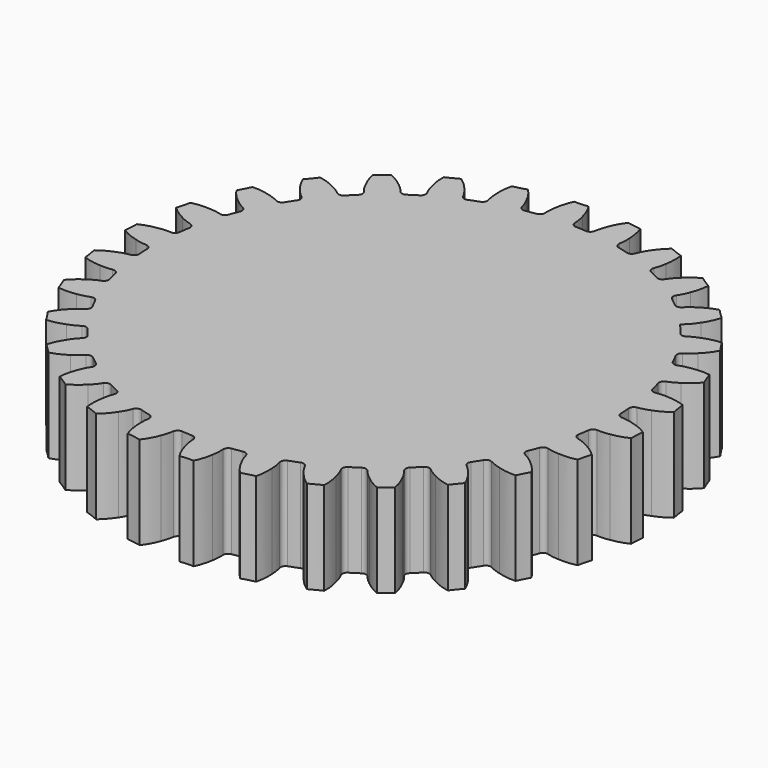
from build123d import *

# Parameters (mm, degrees)
F1_DEPTH = 19.05
F2_COUNT = 30
F4_R     = 1.016


with BuildPart() as f1:
    # F0 (on Top) → F1 (new body)
    with BuildSketch(Plane.XY):
        with BuildLine():
            ThreePointArc((-5.3628156149, 47.1048083691), (-31.5703698192, -35.3685525897), (47.4091, 0))
            ThreePointArc((47.4091, 0), (33.6678157242, 33.3781507453), (0.4096443185, 47.4073301752))
            ThreePointArc((0.4096443185, 47.4073301752), (-2.4812005831, 47.3441274761), (-5.3628156149, 47.1048083691))
        make_face()
        with BuildLine():
            ThreePointArc((-5.3628156149, 47.1048083691), (-2.4812005831, 47.3441274761), (0.4096443185, 47.4073301752))
            ThreePointArc((0.4096443185, 47.4073301752), (0.3511687979, 49.1213355572), (0, 50.8))
            ThreePointArc((0, 50.8), (-0.5741152266, 52.5444861459), (-1.424696856, 54.1721688848))
            ThreePointArc((-1.424696856, 54.1721688848), (-2.8338520024, 54.0731174115), (-4.2456413478, 54.0243294485))
            ThreePointArc((-4.2456413478, 54.0243294485), (-4.9214242267, 52.3166533354), (-5.310045934, 50.5217122847))
            ThreePointArc((-5.310045934, 50.5217122847), (-5.4838227779, 48.8155366066), (-5.3628156149, 47.1048083691))
        make_face()
    extrude(amount=F1_DEPTH)


with BuildPart() as f2_1:
    # F2: instance of F1
    add(f1.part.rotate(Axis((0, 0, 0), (0, 0, -1)), 1 * 360 / F2_COUNT))


with BuildPart() as f2_2:
    # F2: instance of F1
    add(f1.part.rotate(Axis((0, 0, 0), (0, 0, -1)), 2 * 360 / F2_COUNT))


with BuildPart() as f2_3:
    # F2: instance of F1
    add(f1.part.rotate(Axis((0, 0, 0), (0, 0, -1)), 3 * 360 / F2_COUNT))


with BuildPart() as f2_4:
    # F2: instance of F1
    add(f1.part.rotate(Axis((0, 0, 0), (0, 0, -1)), 4 * 360 / F2_COUNT))


with BuildPart() as f2_5:
    # F2: instance of F1
    add(f1.part.rotate(Axis((0, 0, 0), (0, 0, -1)), 5 * 360 / F2_COUNT))


with BuildPart() as f2_6:
    # F2: instance of F1
    add(f1.part.rotate(Axis((0, 0, 0), (0, 0, -1)), 6 * 360 / F2_COUNT))


with BuildPart() as f2_7:
    # F2: instance of F1
    add(f1.part.rotate(Axis((0, 0, 0), (0, 0, -1)), 7 * 360 / F2_COUNT))


with BuildPart() as f2_8:
    # F2: instance of F1
    add(f1.part.rotate(Axis((0, 0, 0), (0, 0, -1)), 8 * 360 / F2_COUNT))


with BuildPart() as f2_9:
    # F2: instance of F1
    add(f1.part.rotate(Axis((0, 0, 0), (0, 0, -1)), 9 * 360 / F2_COUNT))


with BuildPart() as f2_10:
    # F2: instance of F1
    add(f1.part.rotate(Axis((0, 0, 0), (0, 0, -1)), 10 * 360 / F2_COUNT))


with BuildPart() as f2_11:
    # F2: instance of F1
    add(f1.part.rotate(Axis((0, 0, 0), (0, 0, -1)), 11 * 360 / F2_COUNT))


with BuildPart() as f2_12:
    # F2: instance of F1
    add(f1.part.rotate(Axis((0, 0, 0), (0, 0, -1)), 12 * 360 / F2_COUNT))


with BuildPart() as f2_13:
    # F2: instance of F1
    add(f1.part.rotate(Axis((0, 0, 0), (0, 0, -1)), 13 * 360 / F2_COUNT))


with BuildPart() as f2_14:
    # F2: instance of F1
    add(f1.part.rotate(Axis((0, 0, 0), (0, 0, -1)), 14 * 360 / F2_COUNT))


with BuildPart() as f2_15:
    # F2: instance of F1
    add(f1.part.rotate(Axis((0, 0, 0), (0, 0, -1)), 15 * 360 / F2_COUNT))


with BuildPart() as f2_16:
    # F2: instance of F1
    add(f1.part.rotate(Axis((0, 0, 0), (0, 0, -1)), 16 * 360 / F2_COUNT))


with BuildPart() as f2_17:
    # F2: instance of F1
    add(f1.part.rotate(Axis((0, 0, 0), (0, 0, -1)), 17 * 360 / F2_COUNT))


with BuildPart() as f2_18:
    # F2: instance of F1
    add(f1.part.rotate(Axis((0, 0, 0), (0, 0, -1)), 18 * 360 / F2_COUNT))


with BuildPart() as f2_19:
    # F2: instance of F1
    add(f1.part.rotate(Axis((0, 0, 0), (0, 0, -1)), 19 * 360 / F2_COUNT))


with BuildPart() as f2_20:
    # F2: instance of F1
    add(f1.part.rotate(Axis((0, 0, 0), (0, 0, -1)), 20 * 360 / F2_COUNT))


with BuildPart() as f2_21:
    # F2: instance of F1
    add(f1.part.rotate(Axis((0, 0, 0), (0, 0, -1)), 21 * 360 / F2_COUNT))


with BuildPart() as f2_22:
    # F2: instance of F1
    add(f1.part.rotate(Axis((0, 0, 0), (0, 0, -1)), 22 * 360 / F2_COUNT))


with BuildPart() as f2_23:
    # F2: instance of F1
    add(f1.part.rotate(Axis((0, 0, 0), (0, 0, -1)), 23 * 360 / F2_COUNT))


with BuildPart() as f2_24:
    # F2: instance of F1
    add(f1.part.rotate(Axis((0, 0, 0), (0, 0, -1)), 24 * 360 / F2_COUNT))


with BuildPart() as f2_25:
    # F2: instance of F1
    add(f1.part.rotate(Axis((0, 0, 0), (0, 0, -1)), 25 * 360 / F2_COUNT))


with BuildPart() as f2_26:
    # F2: instance of F1
    add(f1.part.rotate(Axis((0, 0, 0), (0, 0, -1)), 26 * 360 / F2_COUNT))


with BuildPart() as f2_27:
    # F2: instance of F1
    add(f1.part.rotate(Axis((0, 0, 0), (0, 0, -1)), 27 * 360 / F2_COUNT))


with BuildPart() as f2_28:
    # F2: instance of F1
    add(f1.part.rotate(Axis((0, 0, 0), (0, 0, -1)), 28 * 360 / F2_COUNT))


with BuildPart() as f2_29:
    # F2: instance of F1
    add(f1.part.rotate(Axis((0, 0, 0), (0, 0, -1)), 29 * 360 / F2_COUNT))


with BuildPart() as f1_1:
    add(f1.part)

    # F3: union F2_1, F2_2, F2_4, F2_3, F2_6, F2_5, F2_7, F2_8, F2_9, F2_10, F2_11, F2_12, F2_13, F2_14, F2_16, F2_17, F2_15, F2_18, F2_19, F2_20, F2_21, F2_22, F2_23, F2_24, F2_25, F2_26, F2_27, F2_28, F2_29
    add(f2_1.part)
    add(f2_2.part)
    add(f2_4.part)
    add(f2_3.part)
    add(f2_6.part)
    add(f2_5.part)
    add(f2_7.part)
    add(f2_8.part)
    add(f2_9.part)
    add(f2_10.part)
    add(f2_11.part)
    add(f2_12.part)
    add(f2_13.part)
    add(f2_14.part)
    add(f2_16.part)
    add(f2_17.part)
    add(f2_15.part)
    add(f2_18.part)
    add(f2_19.part)
    add(f2_20.part)
    add(f2_21.part)
    add(f2_22.part)
    add(f2_23.part)
    add(f2_24.part)
    add(f2_25.part)
    add(f2_26.part)
    add(f2_27.part)
    add(f2_28.part)
    add(f2_29.part)

    # F4
    f4_edges = [f1_1.edges().sort_by_distance(p)[0] for p in [
        (-5.362816, 47.104808, 9.525),
        (0.409644, 47.40733, 9.525),
        (-9.455846, 46.456536, 9.525),
        (4.548015, 47.190447, 9.525),
        (10.257231, 46.286196, 9.525),
        (14.260076, 45.213637, 9.525),
        (19.656527, 43.142134, 9.525),
        (23.348903, 41.260774, 9.525),
        (28.196739, 38.112553, 9.525),
        (31.417271, 35.504618, 9.525),
        (38.112553, 28.196739, 9.525),
        (41.260774, 23.348903, 9.525),
        (43.142134, 19.656527, 9.525),
        (45.213637, 14.260076, 9.525),
        (46.286196, 10.257231, 9.525),
        (47.190447, 4.548015, 9.525),
        (47.40733, 0.409644, 9.525),
        (47.104808, -5.362816, 9.525),
        (46.456536, -9.455846, 9.525),
        (44.960463, -15.039266, 9.525),
        (43.475368, -18.90807, 9.525),
        (40.85113, -24.058427, 9.525),
        (38.594119, -27.53392, 9.525),
        (34.956407, -32.026121, 9.525),
        (32.026121, -34.956407, 9.525),
        (27.53392, -38.594119, 9.525),
        (24.058427, -40.85113, 9.525),
        (18.90807, -43.475368, 9.525),
        (15.039266, -44.960463, 9.525),
        (9.455846, -46.456536, 9.525),
        (5.362816, -47.104808, 9.525),
        (-0.409644, -47.40733, 9.525),
        (-4.548015, -47.190447, 9.525),
        (-10.257231, -46.286196, 9.525),
        (-14.260076, -45.213637, 9.525),
        (-19.656527, -43.142134, 9.525),
        (-23.348903, -41.260774, 9.525),
        (-28.196739, -38.112553, 9.525),
        (-31.417271, -35.504618, 9.525),
        (-35.504618, -31.417271, 9.525),
        (-38.112553, -28.196739, 9.525),
        (-41.260774, -23.348903, 9.525),
        (-43.142134, -19.656527, 9.525),
        (-45.213637, -14.260076, 9.525),
        (-46.286196, -10.257231, 9.525),
        (-47.190447, -4.548015, 9.525),
        (-47.40733, -0.409644, 9.525),
        (-47.104808, 5.362816, 9.525),
        (-46.456536, 9.455846, 9.525),
        (-44.960463, 15.039266, 9.525),
        (-43.475368, 18.90807, 9.525),
        (-40.85113, 24.058427, 9.525),
        (-38.594119, 27.53392, 9.525),
        (-34.956407, 32.026121, 9.525),
        (-32.026121, 34.956407, 9.525),
        (-27.53392, 38.594119, 9.525),
        (-24.058427, 40.85113, 9.525),
        (-18.90807, 43.475368, 9.525),
        (-15.039266, 44.960463, 9.525),
    ]]
    fillet(f4_edges, radius=F4_R)


solid = f1_1.part
